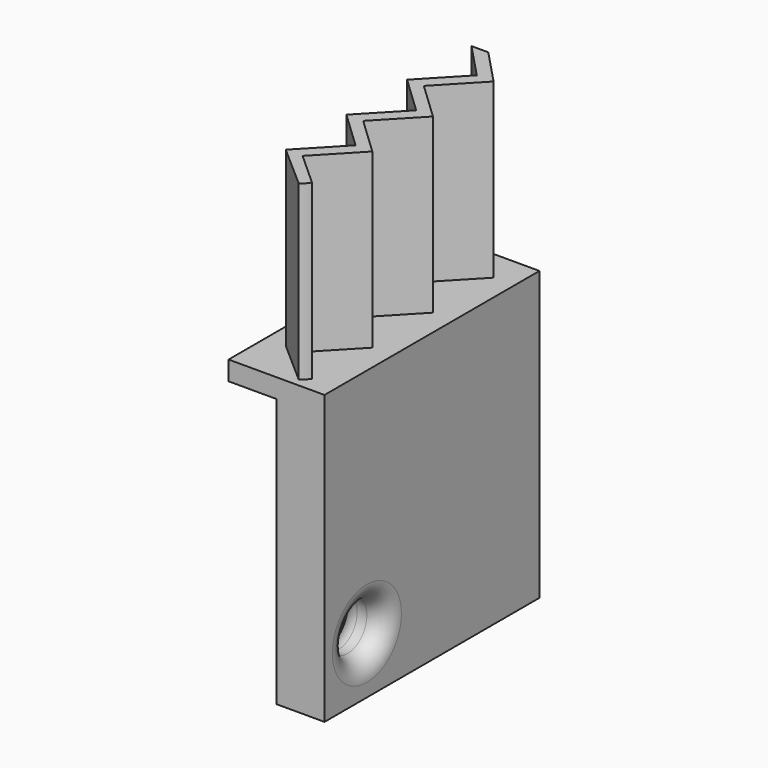
from build123d import *

# Parameters (mm, degrees)
F0_W     = 5
F0_H     = 28
F1_DEPTH = 14
F3_DEPTH = 18
F4_R     = 2.5
F5_DEPTH = 5
F6_R     = 2


# Not quite as in the source:
# - a feature names something its author has since deleted; it is built from what else it names


with BuildPart() as f1:
    # F0 (on Front) → F1 (new body, symmetric)
    with BuildSketch(Plane.XZ):
        Polygon((3.75, 8.5), (-6.25, 8.5), (-6.25, 6.5), (-1.25, 6.5), (3.75, 6.5), align=None)
        with Locations((1.25, -7.5)):
            Rectangle(F0_W, F0_H)
    extrude(amount=F1_DEPTH, both=True)

    # F2 (on face) → F3 (join)
    with BuildSketch(Plane.XY.offset(8.5)):
        with BuildLine():
            Line((-1.9743843018, 14.4904378137), (-3.7243843018, 14.4904378137))
            Line((-3.7243843018, 14.4904378137), (-0.1705003797, 10.7404378137))
            Line((-0.1705003797, 10.7404378137), (-4.1205003797, 6.5904378137))
            Line((-4.1205003797, 6.5904378137), (-0.1705003797, 2.8404378137))
            Line((-0.1705003797, 2.8404378137), (-4.1205003797, -1.3095621863))
            Line((-4.1205003797, -1.3095621863), (-0.1705003797, -5.0595621863))
            Line((-0.1705003797, -5.0595621863), (-4.1205003797, -9.2095621863))
            Line((-4.1205003797, -9.2095621863), (0.4322179562, -13.2100868422))
            ThreePointArc((0.4322179562, -13.2100868422), (0.838165637, -12.8418212057), (1.1682262547, -12.4042448269))
            Line((1.1682262547, -12.4042448269), (-2.3705003797, -9.2095621863))
            Line((-2.3705003797, -9.2095621863), (1.5794996203, -5.0595621863))
            Line((1.5794996203, -5.0595621863), (-2.3705003797, -1.3095621863))
            Line((-2.3705003797, -1.3095621863), (1.5794996203, 2.8404378137))
            Line((1.5794996203, 2.8404378137), (-2.3705003797, 6.5904378137))
            Line((-2.3705003797, 6.5904378137), (1.5794996203, 10.7404378137))
            Line((1.5794996203, 10.7404378137), (-1.9743843018, 14.4904378137))
        make_face()
    extrude(amount=F3_DEPTH)

    # F4 (on face) → F5 (cut, symmetric)
    with BuildSketch(Plane(origin=(-1.25, 0, 0), x_dir=(0, -1, 0), z_dir=(-1, 0, 0))):
        with Locations((8.4821127024, -15.6142489255)):
            Circle(F4_R)
    extrude(amount=F5_DEPTH, both=True, mode=Mode.SUBTRACT)

    # F6
    f6_edges = [f1.edges().sort_by_distance(p)[0] for p in [
        (3.75, -5.982113, -15.614249),
        (-1.25, -5.982113, -15.614249),
    ]]
    fillet(f6_edges, radius=F6_R)


solid = f1.part
